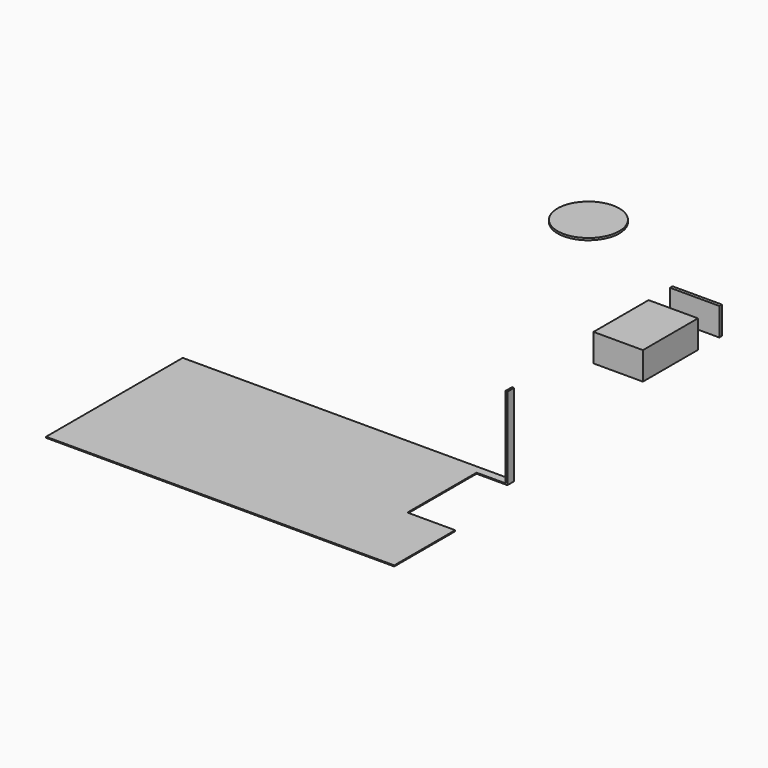
from build123d import *

# Parameters (mm, degrees)
F0_W     = 1200
F0_H     = 77.1629333496
F1_DEPTH = 25
F0_H_2   = 1672.8370666504
F2_DEPTH = 675
F0_W_2   = 50
F0_H_3   = 200
F3_DEPTH = 2000
F4_R     = 750
F5_DEPTH = 50


with BuildPart() as f1:
    # F0 (on Top) → F1 (new body)
    with BuildSketch(Plane.XY):
        with Locations((2126.1950492859, -531.2530517578)):
            Rectangle(F0_W, F0_H)
    extrude(amount=F1_DEPTH)


with BuildPart() as f1b:
    # F0 (on Top) → F1, piece 2 (new body)
    with BuildSketch(Plane.XY):
        with Locations((2126.1950492859, -2056.2530517578)):
            Rectangle(F0_W, F0_H_2)
    extrude(amount=F1_DEPTH)


with BuildPart() as f1c:
    # F0 (on Top) → F1, piece 3 (new body)
    with BuildSketch(Plane.XY):
        Polygon((-2573.8049507141, -11769.8345184326), (3786.1950492859, -11769.8345184326), (3786.1950492859, -9919.8345184326), (2626.1950492859, -9919.8345184326), (2626.1950492859, -7819.8345184326), (3326.1950492859, -7819.8345184326), (3326.1950492859, -7619.8345184326), (-4673.8049507141, -7619.8345184326), (-4673.8049507141, -11769.8345184326), align=None)
    extrude(amount=F1_DEPTH)


with BuildPart() as f2:
    # F0 (on Top) → F2 (new body)
    with BuildSketch(Plane.XY):
        with Locations((2126.1950492859, -2056.2530517578)):
            Rectangle(F0_W, F0_H_2)
    extrude(amount=F2_DEPTH)


with BuildPart() as f2b:
    # F0 (on Top) → F2, piece 2 (new body)
    with BuildSketch(Plane.XY):
        with Locations((2126.1950492859, -531.2530517578)):
            Rectangle(F0_W, F0_H)
    extrude(amount=F2_DEPTH)


with BuildPart() as f3:
    # F0 (on Top) → F3 (new body)
    with BuildSketch(Plane.XY):
        with Locations((3351.1950492859, -7719.8345184326)):
            Rectangle(F0_W_2, F0_H_3)
    extrude(amount=F3_DEPTH)


with BuildPart() as f5:
    # F4 (on face) → F5 (new body)
    with BuildSketch(Plane.XY.offset(25)):
        with Locations((-2147.2208499908, 1545.1865196228)):
            Circle(F4_R)
    extrude(amount=F5_DEPTH)


solid = Compound([f1.part, f1b.part, f1c.part, f2.part, f2b.part, f3.part, f5.part])
